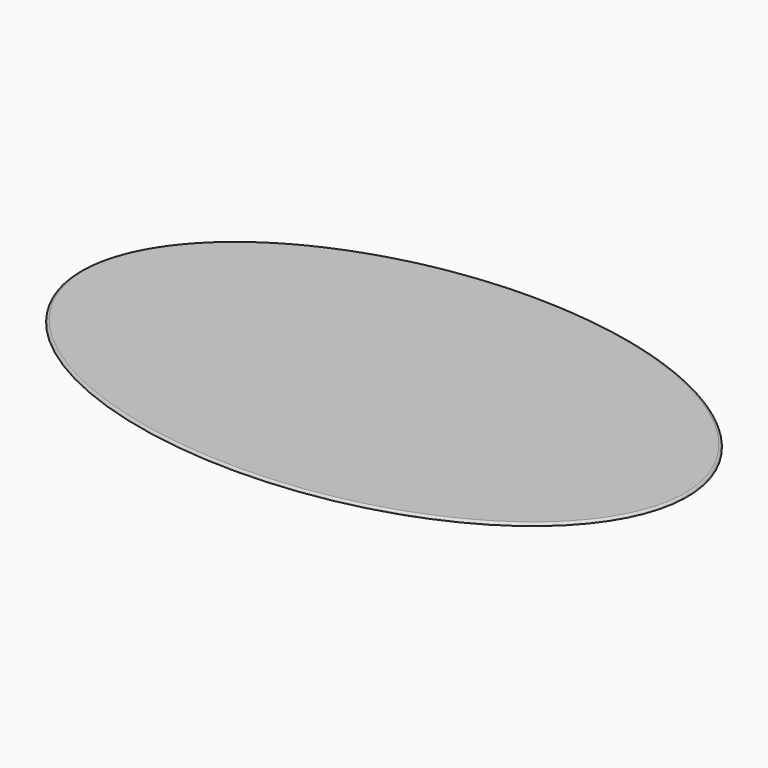
from build123d import *

# Parameters (mm, degrees)
F1_DEPTH = 3
F2_R     = 2.9999
F4_DEPTH = 2


# Not quite as in the source:
# - a fillet or chamfer is up to 0.001 mm smaller than in the source, because OpenCascade refuses the exact size


with BuildPart() as f1:
    # F0 (on Top) → F1 (new body)
    with BuildSketch(Plane.XY):
        with BuildLine():
            add(Edge.make_bspline(
                [(-372.5, 0), (-372.5, -397.1072886513), (186.25, -198.5536443257), (745, 0), (186.25, 198.5536443257), (-372.5, 397.1072886513), (-372.5, 0)],
                knots=[0, 0, 0, 2.0943951024, 2.0943951024, 4.1887902048, 4.1887902048, 6.2831853072, 6.2831853072, 6.2831853072], degree=2, weights=[1, 0.5, 1, 0.5, 1, 0.5, 1]))
        make_face()
    extrude(amount=F1_DEPTH)

    # F2 (radius 3 in the source; OpenCascade refuses exactly that, so slightly less here)
    f2_edges = [f1.edges().sort_by_distance(p)[0] for p in [
        (372.5, -3e-06, 3),
    ]]
    fillet(f2_edges, radius=F2_R)

    # F3 (on face) → F4 (join)
    with BuildSketch(Plane(origin=(0, 0, 0), x_dir=(1, 0, 0), z_dir=(0, 0, -1))):
        with BuildLine():
            add(Edge.make_bspline(
                [(-355, 0), (-355, -366.7963995189), (177.5, -183.3981997594), (710, 0), (177.5, 183.3981997594), (-355, 366.7963995189), (-355, 0)],
                knots=[0, 0, 0, 2.0943951024, 2.0943951024, 4.1887902048, 4.1887902048, 6.2831853072, 6.2831853072, 6.2831853072], degree=2, weights=[1, 0.5, 1, 0.5, 1, 0.5, 1]))
        make_face()
    extrude(amount=F4_DEPTH)


solid = f1.part
